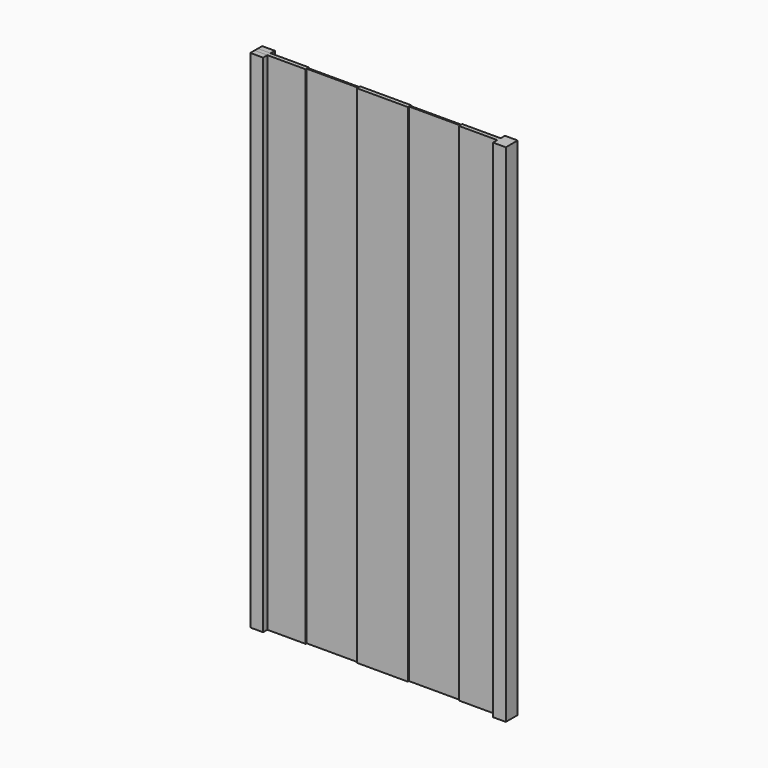
from build123d import *

# Parameters (mm, degrees)
F0_W     = 5
F0_H     = 198
F1_DEPTH = 2.9
F0_W_2   = 15
F2_DEPTH = 0.8
F0_W_3   = 20
F3_DEPTH = 0.3


with BuildPart() as f1:
    # F0 (on Front) → F1 (new body, symmetric)
    with BuildSketch(Plane.XZ):
        with Locations((47.5, 0)):
            Rectangle(F0_W, F0_H)
    extrude(amount=F1_DEPTH, both=True)

    # F0 (on Front) → F2 (join, symmetric)
    with BuildSketch(Plane.XZ):
        with Locations((37.5, 0)):
            Rectangle(F0_W_2, F0_H)
    extrude(amount=F2_DEPTH, both=True)


with BuildPart() as f1b:
    # F0 (on Front) → F1, piece 2 (new body, symmetric)
    with BuildSketch(Plane.XZ):
        with Locations((-47.5, 0)):
            Rectangle(F0_W, F0_H)
    extrude(amount=F1_DEPTH, both=True)


with BuildPart() as f2:
    # F0 (on Front) → F2, piece 2 (new body, symmetric)
    with BuildSketch(Plane.XZ):
        Rectangle(F0_W_3, F0_H)
    extrude(amount=F2_DEPTH, both=True)


with BuildPart() as f2b:
    # F0 (on Front) → F2, piece 3 (new body, symmetric)
    with BuildSketch(Plane.XZ):
        with Locations((-47.5, 0)):
            Rectangle(F0_W, F0_H)
        with Locations((-37.5, 0)):
            Rectangle(F0_W_2, F0_H)
    extrude(amount=F2_DEPTH, both=True)


with BuildPart() as f3:
    # F0 (on Front) → F3 (new body, symmetric)
    with BuildSketch(Plane.XZ):
        with Locations((-20, 0)):
            Rectangle(F0_W_3, F0_H)
    extrude(amount=F3_DEPTH, both=True)


with BuildPart() as f3b:
    # F0 (on Front) → F3, piece 2 (new body, symmetric)
    with BuildSketch(Plane.XZ):
        with Locations((20, 0)):
            Rectangle(F0_W_3, F0_H)
    extrude(amount=F3_DEPTH, both=True)


solid = Compound([f1.part, f1b.part, f2.part, f2b.part, f3.part, f3b.part])
